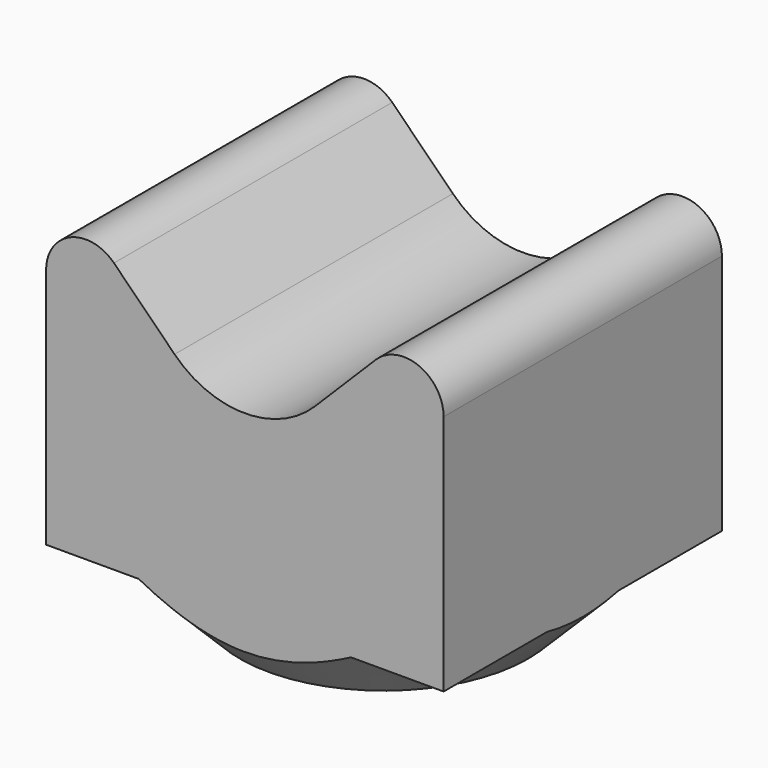
from build123d import *

# Parameters (mm, degrees)
F1_DEPTH = 11.1125
F2_R     = 2.54
F3_R     = 2.4765
F4_DEPTH = 5.08
F5_W     = 25.4
F5_H     = 22.225
F5_R     = 7.9375
F6_DEPTH = 3.81


# Not quite as in the source:
# - a fillet or chamfer that OpenCascade refuses, or shapes differently, is made with other operations: its cross-section is extruded or revolved along the edge and cut away or added


with BuildPart() as f1:
    # F0 (on Front) → F1 (new body, symmetric)
    with BuildSketch(Plane.XZ):
        Polygon((-4.490128064, 4.490128064), (-12.7, 12.7), (-12.7, -12.7), (12.7, -12.7), (12.7, 12.7), (4.4901280734, 4.4901280734), (0, 0), align=None)
        with BuildLine():
            ThreePointArc((4.4901280734, 4.4901280734), (6.6e-09, 2.6302561211), (-4.490128064, 4.490128064))
            Line((-4.490128064, 4.490128064), (0, 0))
            Line((0, 0), (4.4901280734, 4.4901280734))
        make_face()
    extrude(amount=F1_DEPTH, both=True)

    # F2
    f2_edges = [f1.edges().sort_by_distance(p)[0] for p in [
        (12.7, 0, 12.7),
        (-12.7, 0, 12.7),
    ]]
    fillet(f2_edges, radius=F2_R)

    # F3 (on face) → F4 (cut)
    with BuildSketch(Plane(origin=(0, 0, -12.7), x_dir=(1, 0, 0), z_dir=(0, 0, -1))):
        Circle(F3_R)
    extrude(amount=-F4_DEPTH, mode=Mode.SUBTRACT)

    # F5 (on face) → F6 (cut)
    with BuildSketch(Plane(origin=(0, 0, -12.7), x_dir=(1, 0, 0), z_dir=(0, 0, -1))):
        Rectangle(F5_W, F5_H)
        Circle(F5_R, mode=Mode.SUBTRACT)
    extrude(amount=-F6_DEPTH, mode=Mode.SUBTRACT)

    # F7: chamfer of 5.08 on 1 edges, made by hand


with BuildPart() as f7_tool2:
    # F7_s3 → F7_t4 (revolve)
    with BuildSketch(Plane.XZ):
        Polygon((13.0175, -8.89), (7.9375, -13.97), (7.9375, -8.89), align=None)
    revolve(axis=Axis((0, 0, -8.89), (0, 0, -1)))

    split(bisect_by=Plane.XZ.offset(-11.1125), keep=Keep.TOP)

    split(bisect_by=Plane.XZ.offset(11.1125), keep=Keep.BOTTOM)

    split(bisect_by=Plane.YZ.offset(12.7), keep=Keep.BOTTOM)

    split(bisect_by=Plane.YZ.offset(-12.7), keep=Keep.TOP)

    split(bisect_by=Plane.XY.offset(-12.7), keep=Keep.TOP)


with BuildPart() as f1_1:
    add(f1.part)

    # F7_t1: union F7_tool2
    add(f7_tool2.part)


solid = f1_1.part
